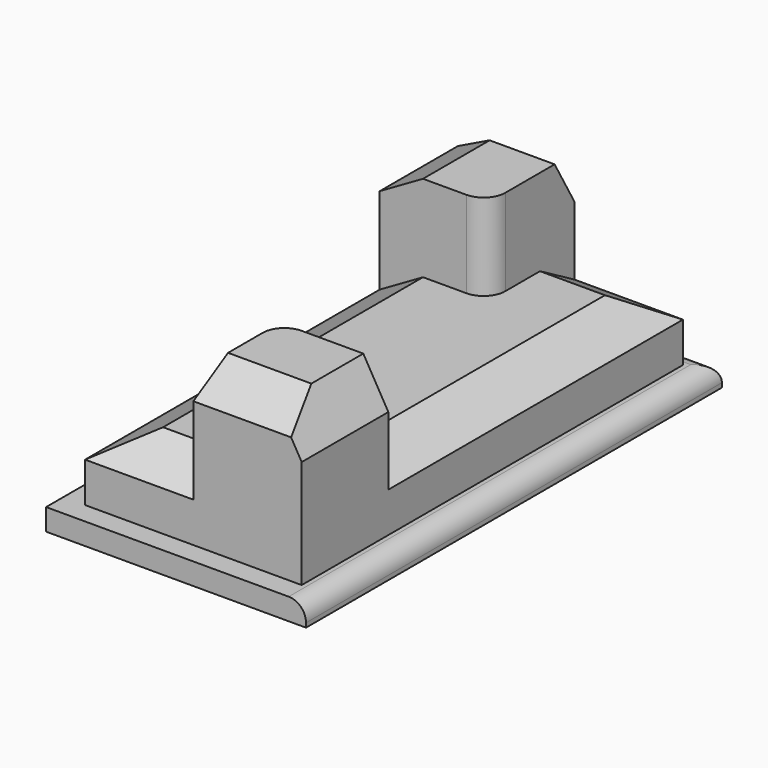
from build123d import *

# Parameters (mm, degrees)
F0_W        = 76.2
F0_H        = 152.4
F1_DEPTH    = 6.35
F2_DEPTH    = 25.4
F0_W_2      = 31.75
F0_H_2      = 31.75
F3_DEPTH    = 50.8
F4_C1_SIZE2 = 12.7
F4_C1_SIZE  = 7.3323484187
F4_C2_SIZE2 = 12.7
F4_C2_SIZE  = 7.3323484187
F4_C3_SIZE2 = 7.3323484187
F4_C3_SIZE  = 12.7
F4_C4_SIZE2 = 12.7
F4_C4_SIZE  = 7.3323484187
F4_C5_SIZE2 = 7.3323484187
F4_C5_SIZE  = 12.7
F4_C6_SIZE2 = 7.3323484187
F4_C6_SIZE  = 12.7
F4_C7_SIZE2 = 7.3323484187
F4_C7_SIZE  = 12.7
F4_C8_SIZE2 = 12.7
F4_C8_SIZE  = 7.3323484187
F5_R        = 6.35
F6_R        = 5.08


with BuildPart() as f1:
    # F0 (on Top) → F1 (new body)
    with BuildSketch(Plane.XY):
        with Locations((2.3026284762, 11.2662552908)):
            Rectangle(F0_W, F0_H)
        Polygon((-29.4473715238, 49.3662552908), (-29.4473715238, 81.1162552908), (2.3026284762, 81.1162552908), (34.0526284762, 81.1162552908), (34.0526284762, -26.8337447092), (34.0526284762, -58.5837447092), (2.3026284762, -58.5837447092), (-29.4473715238, -58.5837447092), align=None, mode=Mode.SUBTRACT)
    extrude(amount=F1_DEPTH)

    # F0 (on Top) → F2 (join)
    with BuildSketch(Plane.XY):
        Polygon((34.0526284762, 81.1162552908), (2.3026284762, 81.1162552908), (2.3026284762, 49.3662552908), (-29.4473715238, 49.3662552908), (-29.4473715238, -58.5837447092), (2.3026284762, -58.5837447092), (2.3026284762, -26.8337447092), (34.0526284762, -26.8337447092), align=None)
    extrude(amount=F2_DEPTH)

    # F0 (on Top) → F3 (join)
    with BuildSketch(Plane.XY):
        with Locations((-13.5723715238, 65.2412552908)):
            Rectangle(F0_W_2, F0_H_2)
        with Locations((18.1776284762, -42.7087447092)):
            Rectangle(F0_W_2, F0_H_2)
    extrude(amount=F3_DEPTH)

    # F4: chamfer of 12.7 x 7.3323484187 on 8 edges, made by hand

    # F4_c1
    f4_c1_edges = [f1.edges().sort_by_distance(p)[0] for p in [
        (-13.5723715238, -58.5837447092, 25.4),
    ]]
    f4_c1_side = f1.faces().sort_by_distance((-13.5723715238, -58.5837447092, 25.2533530316))[0]
    chamfer(f4_c1_edges, length=F4_C1_SIZE, length2=F4_C1_SIZE2, reference=f4_c1_side)

    # F4_c2
    f4_c2_edges = [f1.edges().sort_by_distance(p)[0] for p in [
        (18.1776284762, -58.5837447092, 50.8),
    ]]
    f4_c2_side = f1.faces().sort_by_distance((18.1776284762, -58.5837447092, 50.6533530316))[0]
    chamfer(f4_c2_edges, length=F4_C2_SIZE, length2=F4_C2_SIZE2, reference=f4_c2_side)

    # F4_c3
    f4_c3_edges = [f1.edges().sort_by_distance(p)[0] for p in [
        (34.0526284762, -36.3587447092, 50.8),
    ]]
    f4_c3_side = f1.faces().sort_by_distance((34.0526284762, -36.3587447092, 50.6533530316))[0]
    chamfer(f4_c3_edges, length=F4_C3_SIZE, length2=F4_C3_SIZE2, reference=f4_c3_side)

    # F4_c4
    f4_c4_edges = [f1.edges().sort_by_distance(p)[0] for p in [
        (18.1776284762, 81.1162552908, 25.4),
    ]]
    f4_c4_side = f1.faces().sort_by_distance((18.1776284762, 81.1162552908, 25.2533530316))[0]
    chamfer(f4_c4_edges, length=F4_C4_SIZE, length2=F4_C4_SIZE2, reference=f4_c4_side)

    # F4_c5
    f4_c5_edges = [f1.edges().sort_by_distance(p)[0] for p in [
        (-29.4473715238, 1.7412552908, 25.4),
    ]]
    f4_c5_side = f1.faces().sort_by_distance((-29.3007245555, 1.7412552908, 25.4))[0]
    chamfer(f4_c5_edges, length=F4_C5_SIZE, length2=F4_C5_SIZE2, reference=f4_c5_side)

    # F4_c6
    f4_c6_edges = [f1.edges().sort_by_distance(p)[0] for p in [
        (34.0526284762, 20.7912552908, 25.4),
    ]]
    f4_c6_side = f1.faces().sort_by_distance((33.9059815078, 20.7912552908, 25.4))[0]
    chamfer(f4_c6_edges, length=F4_C6_SIZE, length2=F4_C6_SIZE2, reference=f4_c6_side)

    # F4_c7
    f4_c7_edges = [f1.edges().sort_by_distance(p)[0] for p in [
        (-29.4473715238, 65.2412552908, 50.8),
    ]]
    f4_c7_side = f1.faces().sort_by_distance((-29.3007245555, 65.2412552908, 50.8))[0]
    chamfer(f4_c7_edges, length=F4_C7_SIZE, length2=F4_C7_SIZE2, reference=f4_c7_side)

    # F4_c8
    f4_c8_edges = [f1.edges().sort_by_distance(p)[0] for p in [
        (-7.2223715238, 81.1162552908, 50.8),
    ]]
    f4_c8_side = f1.faces().sort_by_distance((-7.2223715238, 80.9696083224, 50.8))[0]
    chamfer(f4_c8_edges, length=F4_C8_SIZE, length2=F4_C8_SIZE2, reference=f4_c8_side)

    # F5
    f5_edges = [f1.edges().sort_by_distance(p)[0] for p in [
        (2.302628, 49.366255, 38.1),
        (2.302628, -26.833745, 38.1),
    ]]
    fillet(f5_edges, radius=F5_R)

    # F6
    f6_edges = [f1.edges().sort_by_distance(p)[0] for p in [
        (2.302628, 87.466255, 6.35),
        (40.402628, 11.266255, 6.35),
    ]]
    fillet(f6_edges, radius=F6_R)


solid = f1.part
